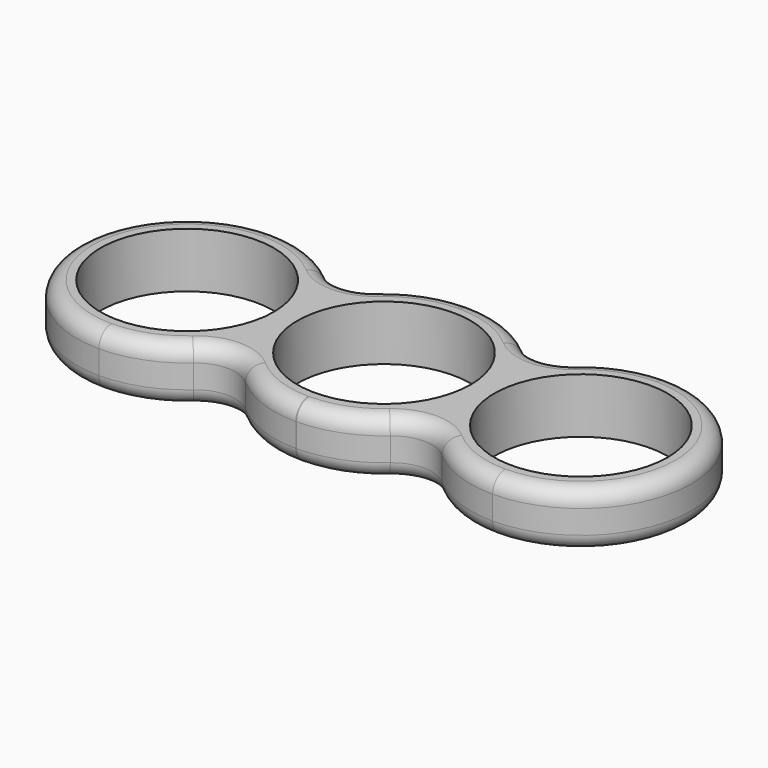
from build123d import *

# Parameters (mm, degrees)
F0_R     = 11
F1_DEPTH = 7
F2_R     = 2


with BuildPart() as f1:
    # F0 (on Top) → F1 (new body)
    with BuildSketch(Plane.XY):
        with BuildLine():
            Line((0, 13.7662742315), (-0.2493512723, 13.7662742315))
            ThreePointArc((-0.2493512723, 13.7662742315), (-5.0736160165, 12.8629735533), (-9.289676891, 10.3501438459))
            ThreePointArc((-9.289676891, 10.3501438459), (-12.5626774859, 9.1299474023), (-15.8357192501, 10.3500334095))
            ThreePointArc((-15.8357192501, 10.3500334095), (-20.1098378601, 12.8844415671), (-25, 13.7662742315))
            ThreePointArc((-25, 13.7662742315), (-39, -0.2337257685), (-25, -14.2337257685))
            ThreePointArc((-25, -14.2337257685), (-20.06914371, -13.3366335009), (-15.7702181307, -10.7603266183))
            ThreePointArc((-15.7702181307, -10.7603266183), (-12.4738019663, -9.5198039469), (-9.1773880082, -10.760332481))
            ThreePointArc((-9.1773880082, -10.760332481), (-4.9029741478, -13.3274190585), (0, -14.2337257685))
            Line((0, -14.2337257685), (0.1052322339, -14.2337257685))
            ThreePointArc((0.1052322339, -14.2337257685), (4.9841023878, -13.3365164219), (9.2438147586, -10.7942321916))
            ThreePointArc((9.2438147586, -10.7942321916), (12.5263567285, -9.5658106543), (15.8089072394, -10.7942093685))
            ThreePointArc((15.8089072394, -10.7942093685), (20.0932072797, -13.3456815799), (25, -14.2337257685))
            ThreePointArc((25, -14.2337257685), (39, -0.2337257685), (25, 13.7662742315))
            ThreePointArc((25, 13.7662742315), (20.0871666697, 12.8759679224), (15.7991799837, 10.3182840413))
            ThreePointArc((15.7991799837, 10.3182840413), (12.5131691049, 9.0868589734), (9.2271600635, 10.3182889441))
            ThreePointArc((9.2271600635, 10.3182889441), (4.9514751973, 12.8713656379), (0.052616117, 13.7662742315))
            Line((0.052616117, 13.7662742315), (0, 13.7662742315))
        make_face()
        with Locations((-25, -0.2337257685)):
            Circle(F0_R, mode=Mode.SUBTRACT)
        with Locations((0, -0.2337257685)):
            Circle(F0_R, mode=Mode.SUBTRACT)
        with Locations((25, -0.2337257685)):
            Circle(F0_R, mode=Mode.SUBTRACT)
    extrude(amount=F1_DEPTH)

    # F2
    f2_edges = [f1.edges().sort_by_distance(p)[0] for p in [
        (-15.835719, 10.350033, 3.5),
        (-38.118167, 4.656436, 7),
        (-25, -14.233726, 3.5),
        (-38.118167, 4.656436, 0),
        (-15.770218, -10.760327, 3.5),
        (-20.069144, -13.336634, 0),
        (-20.069144, -13.336634, 7),
        (-9.177388, -10.760332, 3.5),
        (-12.473802, -9.519804, 0),
        (-12.473802, -9.519804, 7),
        (0.105232, -14.233726, 3.5),
        (9.243815, -10.794232, 3.5),
        (4.984102, -13.336516, 0),
        (4.984102, -13.336516, 7),
        (15.808907, -10.794209, 3.5),
        (12.526357, -9.565811, 0),
        (12.526357, -9.565811, 7),
        (38.111956, -5.140518, 7),
        (25, 13.766274, 3.5),
        (38.111956, -5.140518, 0),
        (-9.289677, 10.350144, 3.5),
        (-12.562677, 9.129947, 0),
        (-12.562677, 9.129947, 7),
        (-0.249351, 13.766274, 3.5),
        (-5.073616, 12.862974, 0),
        (-5.073616, 12.862974, 7),
        (9.22716, 10.318289, 3.5),
        (0.052616, 13.766274, 3.5),
        (4.951475, 12.871366, 0),
        (4.951475, 12.871366, 7),
        (15.79918, 10.318284, 3.5),
        (12.513169, 9.086859, 0),
        (12.513169, 9.086859, 7),
        (-4.902974, -13.327419, 0),
        (-4.902974, -13.327419, 7),
        (0.052616, -14.233726, 7),
        (20.087167, 12.875968, 7),
        (-0.098368, 13.766274, 7),
        (-0.098368, 13.766274, 0),
        (20.087167, 12.875968, 0),
        (0.052616, -14.233726, 0),
    ]]
    fillet(f2_edges, radius=F2_R)


solid = f1.part
